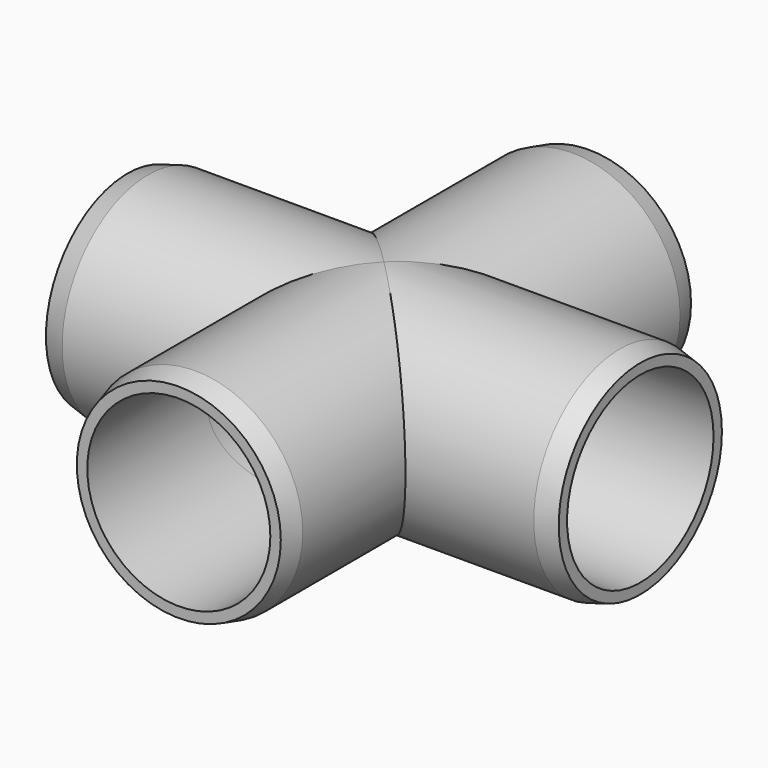
from build123d import *
from build123d import SkipClean  # not in build123d's __all__

# Parameters (mm, degrees)
F0_R          = 24.765
F0_R_2        = 21.082
F1_DEPTH      = 59.055
F2_R          = 24.765
F2_R_2        = 21.082
F3_DEPTH      = 59.055
F4_DEPTH      = 59.0560001
F4_DEPTH_BACK = 59.0560001
F5_DEPTH      = 59.0560001
F5_DEPTH_BACK = 59.0560001
F6_SIZE2      = 1.27
F6_SIZE       = 4.7397045256
F6_2_SIZE2    = 1.27
F6_2_SIZE     = 4.7397045256
F6_3_SIZE2    = 1.27
F6_3_SIZE     = 4.7397045256
F6_4_SIZE2    = 1.27
F6_4_SIZE     = 4.7397045256


# Not quite as in the source:
# - two fillets or chamfers of one size are made in one step


with BuildPart() as f1:
    # F0 (on Front) → F1 (new body, symmetric)
    with BuildSketch(Plane.XZ):
        Circle(F0_R)
        Circle(F0_R_2, mode=Mode.SUBTRACT)
    extrude(amount=F1_DEPTH, both=True)

    # F2 (on Right) → F3 (join, symmetric)
    with BuildSketch(Plane.YZ):
        Circle(F2_R)
        Circle(F2_R_2, mode=Mode.SUBTRACT)
    extrude(amount=F3_DEPTH, both=True)

    # F2 (on Right) → F4 (cut, two sides)
    with BuildSketch(Plane.YZ) as f4_sk:
        Circle(F2_R_2)
    with SkipClean():  # cleaning this boolean's faces spoils the solid; the shape is the same uncleaned
        extrude(amount=F4_DEPTH, mode=Mode.SUBTRACT)
        extrude(f4_sk.sketch, amount=-F4_DEPTH_BACK, mode=Mode.SUBTRACT)

    # F0 (on Front) → F5 (cut, two sides)
    with BuildSketch(Plane.XZ) as f5_sk:
        Circle(F0_R_2)
    extrude(amount=F5_DEPTH, mode=Mode.SUBTRACT)
    extrude(f5_sk.sketch, amount=-F5_DEPTH_BACK, mode=Mode.SUBTRACT)

    # F6
    f6_edges = [f1.edges().sort_by_distance(p)[0] for p in [
        (-59.055, -24.765, 0),
    ]]
    f6_side = f1.faces().sort_by_distance((-29.5275, -24.765, 0))[0]
    chamfer(f6_edges, length=F6_SIZE, length2=F6_SIZE2, reference=f6_side)

    # F6#2
    f6_2_edges = [f1.edges().sort_by_distance(p)[0] for p in [
        (59.055, -24.765, 0),
    ]]
    f6_2_side = f1.faces().sort_by_distance((29.5275, -24.765, 0))[0]
    chamfer(f6_2_edges, length=F6_2_SIZE, length2=F6_2_SIZE2, reference=f6_2_side)

    # F6#3
    f6_3_edges = [f1.edges().sort_by_distance(p)[0] for p in [
        (-24.765, -59.055, 0),
    ]]
    f6_3_side = f1.faces().sort_by_distance((-24.765, -29.5275, 0))[0]
    chamfer(f6_3_edges, length=F6_3_SIZE, length2=F6_3_SIZE2, reference=f6_3_side)

    # F6#4
    f6_4_edges = [f1.edges().sort_by_distance(p)[0] for p in [
        (-24.765, 59.055, 0),
    ]]
    f6_4_side = f1.faces().sort_by_distance((-24.765, 29.5275, 0))[0]
    chamfer(f6_4_edges, length=F6_4_SIZE, length2=F6_4_SIZE2, reference=f6_4_side)


solid = f1.part
